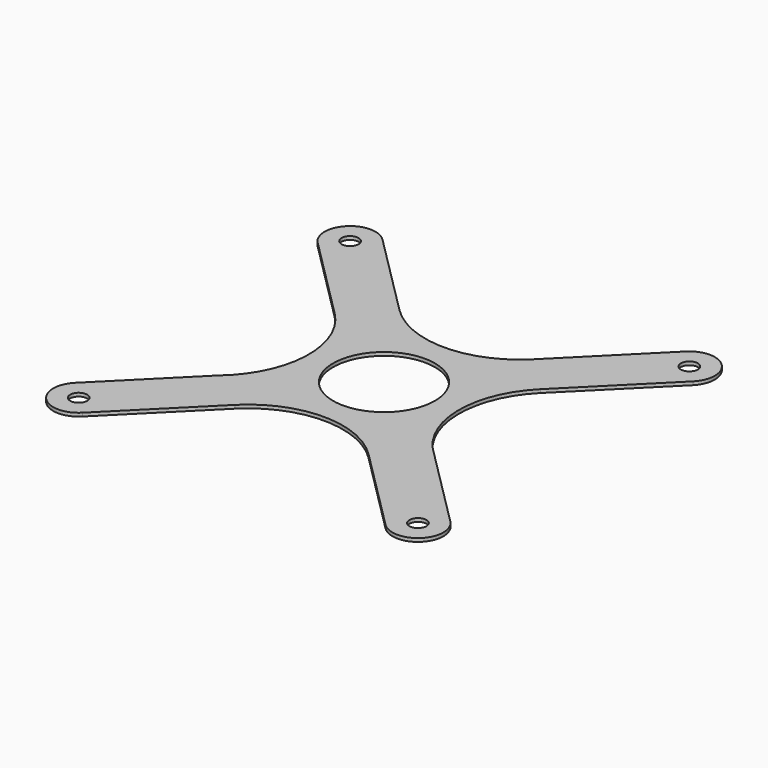
from build123d import *

# Parameters (mm, degrees)
F0_R     = 2.5
F0_R_2   = 15
F1_DEPTH = 1


# Not quite as in the source:
# - ends of sketch curves that miss each other by under 0.0002 mm in the source are joined


with BuildPart() as f1:
    # F0 (on Top) → F1 (new body)
    with BuildSketch(Plane.XY):
        with BuildLine():
            ThreePointArc((11.259775071, 22.0479804919), (-8.4369240701, 13.8893405737), (-28.1336232112, 22.0479804919))
            Line((-28.1336232112, 22.0479804919), (-53.1336232112, 47.0479804919))
            ThreePointArc((-53.1336232112, 47.0479804919), (-63.740224929, 47.0479804919), (-63.740224929, 36.4413787741))
            Line((-63.740224929, 36.4413787741), (-38.740224929, 11.4413787741))
            ThreePointArc((-38.740224929, 11.4413787741), (-30.5775634521, -9.4678572948), (-40.4261190382, -29.6379130271))
            Line((-40.4261190382, -29.6379130271), (-63.7402252241, -52.952019213))
            ThreePointArc((-63.7402252241, -52.952019213), (-63.740225272, -63.5586215688), (-53.1336228682, -63.5586215688))
            Line((-53.1336228682, -63.5586215688), (-28.1336232112, -38.5586212259))
            ThreePointArc((-28.1336232112, -38.5586212259), (-8.4369240701, -30.3999813076), (11.259775071, -38.5586212259))
            Line((11.259775071, -38.5586212259), (36.259775071, -63.5586212259))
            ThreePointArc((36.259775071, -63.5586212259), (46.8663773553, -63.5586217924), (46.8663773553, -52.9520189415))
            Line((46.8663773553, -52.9520189415), (22.9697427144, -29.0553843966))
            ThreePointArc((22.9697427144, -29.0553843966), (13.7059638015, -9.0443706663), (21.8663767888, 11.4413787741))
            Line((21.8663767888, 11.4413787741), (46.8663766102, 36.4413789527))
            ThreePointArc((46.8663766102, 36.4413789527), (46.8663761898, 47.0479798929), (36.25977567, 47.0479798929))
            Line((36.25977567, 47.0479798929), (11.259775071, 22.0479804919))
        make_face()
        with Locations((-58.4369240701, -58.255320367)):
            Circle(F0_R, mode=Mode.SUBTRACT)
        with Locations((41.5630759299, -58.255320367)):
            Circle(F0_R, mode=Mode.SUBTRACT)
        with Locations((-8.4369240701, -8.255320367)):
            Circle(F0_R_2, mode=Mode.SUBTRACT)
        with Locations((-58.4369240701, 41.744679633)):
            Circle(F0_R, mode=Mode.SUBTRACT)
        with Locations((41.5630759299, 41.744679633)):
            Circle(F0_R, mode=Mode.SUBTRACT)
    extrude(amount=F1_DEPTH)


solid = f1.part
